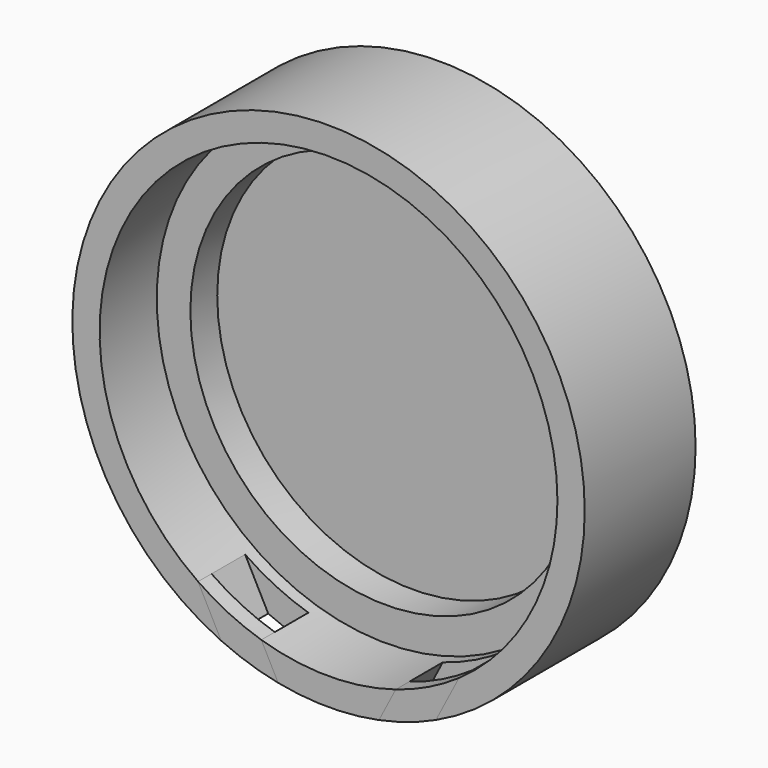
from build123d import *
from build123d import SkipClean  # not in build123d's __all__

# Parameters (mm, degrees)
F0_R     = 6.1
F0_R_2   = 5
F1_DEPTH = 0.8
F2_R     = 6.1
F2_R_2   = 5.45
F3_DEPTH = 2.5
F4_R     = 5.45
F4_R_2   = 4.65
F5_DEPTH = 0.8
F7_DEPTH = 1.4
F9_DEPTH = 0.4


with BuildPart() as f1:
    # F0 (on Front) → F1 (new body)
    with BuildSketch(Plane.XZ):
        Circle(F0_R)
        Circle(F0_R_2, mode=Mode.SUBTRACT)
        Circle(F0_R_2)
    extrude(amount=F1_DEPTH)

    # F2 (on face) → F3 (join)
    with BuildSketch(Plane.XZ.offset(0.8)):
        Circle(F2_R)
        Circle(F2_R_2, mode=Mode.SUBTRACT)
    extrude(amount=F3_DEPTH)

    # F4 (on face) → F5 (join)
    with BuildSketch(Plane.XZ.offset(0.8)):
        Circle(F4_R)
        Circle(F4_R_2, mode=Mode.SUBTRACT)
    extrude(amount=F5_DEPTH)

    # F6 (on face) → F7 (cut)
    with BuildSketch(Plane.XZ.offset(3.3)):
        with BuildLine():
            Line((-1.2, -5.9808026217), (-1.6, -5.2098464469))
            ThreePointArc((-1.6, -5.2098464469), (-2.3813713563, -4.9022005735), (-3.1062049616, -4.4781682345))
            Line((-3.1062049616, -4.4781682345), (-2.555971444, -5.5386830544))
            ThreePointArc((-2.555971444, -5.5386830544), (-1.8909515594, -5.7995087895), (-1.2, -5.9808026217))
        make_face()
        with BuildLine():
            ThreePointArc((3.1062049616, -4.4781682345), (2.3813713563, -4.9022005735), (1.6, -5.2098464469))
            Line((1.6, -5.2098464469), (1.2, -5.9808026217))
            ThreePointArc((1.2, -5.9808026217), (1.8909515594, -5.7995087895), (2.555971444, -5.5386830544))
            Line((2.555971444, -5.5386830544), (3.1062049616, -4.4781682345))
        make_face()
    extrude(amount=-F7_DEPTH, mode=Mode.SUBTRACT)

    # F8 (on face) → F9 (join)
    with BuildSketch(Plane.XZ.offset(3.3)):
        with BuildLine():
            ThreePointArc((-1.6, -5.2098464469), (-2.3813713563, -4.9022005735), (-3.1062049616, -4.4781682345))
            Line((-3.1062049616, -4.4781682345), (-2.555971444, -5.5386830544))
            ThreePointArc((-2.555971444, -5.5386830544), (-1.8909515594, -5.7995087895), (-1.2, -5.9808026217))
            Line((-1.2, -5.9808026217), (-1.6, -5.2098464469))
        make_face()
        with BuildLine():
            Line((2.555971444, -5.5386830544), (3.1062049616, -4.4781682345))
            ThreePointArc((3.1062049616, -4.4781682345), (2.3813713563, -4.9022005735), (1.6, -5.2098464469))
            Line((1.6, -5.2098464469), (1.2, -5.9808026217))
            ThreePointArc((1.2, -5.9808026217), (1.8909515594, -5.7995087895), (2.555971444, -5.5386830544))
        make_face()
    with SkipClean():  # cleaning this boolean's faces spoils the solid; the shape is the same uncleaned
        extrude(amount=-F9_DEPTH)


solid = f1.part
